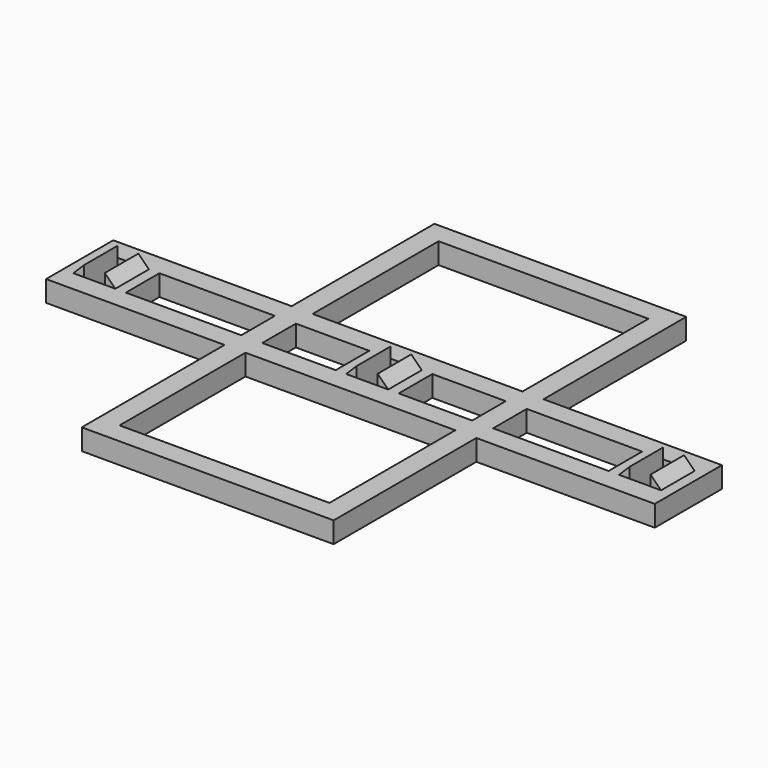
from build123d import *

# Parameters (mm, degrees)
F0_W     = 5
F0_H     = 5
F0_W_2   = 2.5
F0_H_2   = 10
F1_DEPTH = 5
F2_DEPTH = 7.5
F3_SIZE  = 2.49999


# Not quite as in the source:
# - a fillet or chamfer is up to 0.001 mm smaller than in the source, because OpenCascade refuses the exact size
# - a feature names something its author has since deleted; it is built from what else it names


with BuildPart() as f1:
    # F0 (on Top) → F1 (new body)
    with BuildSketch(Plane.XY):
        Polygon((-5, 5), (-2.5, 5), (2.5, 5), (5, 5), (7.5, 5), (25, 5), (25, 10), (-25, 10), (-25, 5), (-7.5, 5), align=None)
        Polygon((-57.5, 5), (-30, 5), (-30, 10), (-72.5, 10), (-72.5, 5), (-70, 5), (-67.5, 5), (-62.5, 5), (-60, 5), align=None)
        Polygon((-30, 10), (-25, 10), (-25, 47.5), (25, 47.5), (25, 10), (30, 10), (30, 52.5), (-30, 52.5), align=None)
        with Locations((-27.5, 7.5)):
            Rectangle(F0_W, F0_H)
        with Locations((-27.5, -7.5)):
            Rectangle(F0_W, F0_H)
        Polygon((-25, -47.5), (-25, -10), (-30, -10), (-30, -52.5), (30, -52.5), (30, -10), (25, -10), (25, -47.5), align=None)
        with Locations((27.5, 7.5)):
            Rectangle(F0_W, F0_H)
        Polygon((30, 10), (30, 5), (57.5, 5), (60, 5), (62.5, 5), (67.5, 5), (70, 5), (72.5, 5), (72.5, 10), align=None)
        with Locations((27.5, -7.5)):
            Rectangle(F0_W, F0_H)
        with Locations((61.25, 0)):
            Rectangle(F0_W_2, F0_H_2)
        with Locations((68.75, 0)):
            Rectangle(F0_W_2, F0_H_2)
        Polygon((2.5, -5), (-2.5, -5), (-5, -5), (-7.5, -5), (-25, -5), (-25, -10), (25, -10), (25, -5), (7.5, -5), (5, -5), align=None)
        with Locations((-3.75, 0)):
            Rectangle(F0_W_2, F0_H_2)
        with Locations((3.75, 0)):
            Rectangle(F0_W_2, F0_H_2)
        Polygon((-30, -10), (-30, -5), (-57.5, -5), (-60, -5), (-62.5, -5), (-67.5, -5), (-70, -5), (-72.5, -5), (-72.5, -10), align=None)
        with Locations((-68.75, 0)):
            Rectangle(F0_W_2, F0_H_2)
        with Locations((-61.25, 0)):
            Rectangle(F0_W_2, F0_H_2)
        with Locations((-71.25, 0)):
            Rectangle(F0_W_2, F0_H_2)
        with Locations((-58.75, 0)):
            Rectangle(F0_W_2, F0_H_2)
        Polygon((57.5, -5), (30, -5), (30, -10), (72.5, -10), (72.5, -5), (70, -5), (67.5, -5), (62.5, -5), (60, -5), align=None)
        with Locations((58.75, 0)):
            Rectangle(F0_W_2, F0_H_2)
        with Locations((71.25, 0)):
            Rectangle(F0_W_2, F0_H_2)
        with Locations((6.25, 0)):
            Rectangle(F0_W_2, F0_H_2)
        with Locations((-6.25, 0)):
            Rectangle(F0_W_2, F0_H_2)
        with Locations((-27.5, 0)):
            Rectangle(F0_W, F0_H_2)
        with Locations((27.5, 0)):
            Rectangle(F0_W, F0_H_2)
    extrude(amount=F1_DEPTH)

    # F0 (on Top) → F2 (join)
    with BuildSketch(Plane.XY):
        with Locations((-68.75, 0)):
            Rectangle(F0_W_2, F0_H_2)
        with Locations((-61.25, 0)):
            Rectangle(F0_W_2, F0_H_2)
        with Locations((-3.75, 0)):
            Rectangle(F0_W_2, F0_H_2)
        with Locations((3.75, 0)):
            Rectangle(F0_W_2, F0_H_2)
        with Locations((61.25, 0)):
            Rectangle(F0_W_2, F0_H_2)
        with Locations((68.75, 0)):
            Rectangle(F0_W_2, F0_H_2)
    extrude(amount=F2_DEPTH)

    # F3 (size 2.5 in the source; OpenCascade refuses exactly that, so slightly less here)
    f3_edges = [f1.edges().sort_by_distance(p)[0] for p in [
        (70, 0, 7.5),
        (60, 0, 7.5),
        (5, 0, 7.5),
        (-5, 0, 7.5),
        (-60, 0, 7.5),
        (-70, 0, 7.5),
    ]]
    chamfer(f3_edges, length=F3_SIZE)


solid = f1.part
